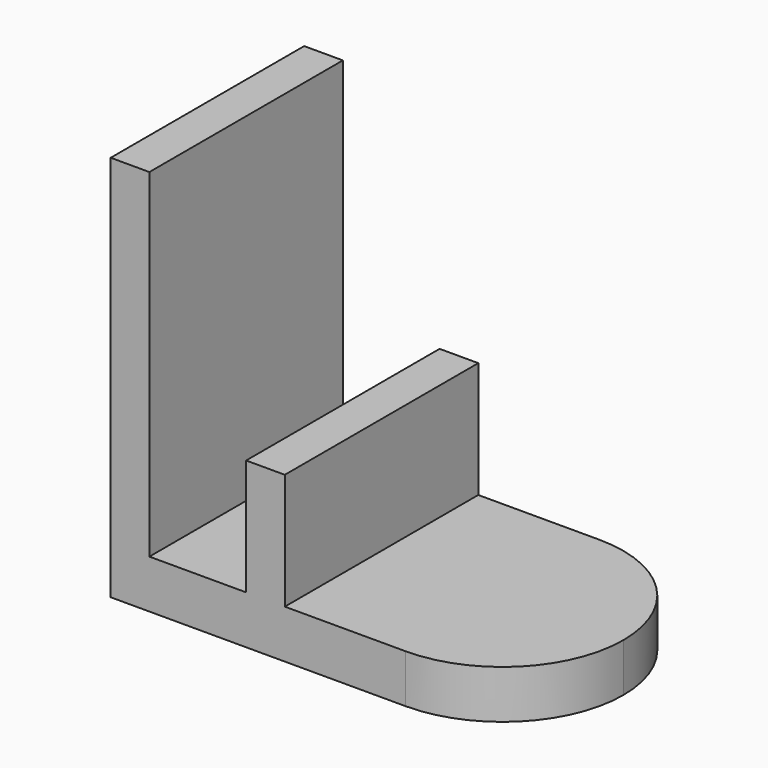
from build123d import *

# Parameters (mm, degrees)
F2_DEPTH = 50
F3_R     = 25
F4_R     = 24.99999


# Not quite as in the source:
# - a fillet or chamfer is up to 0.001 mm smaller than in the source, because OpenCascade refuses the exact size


with BuildPart() as f2:
    # F1 (on face) → F2 (new body)
    with BuildSketch(Plane.XZ):
        Polygon((8, 80), (0, 80), (0, 0), (86, 0), (86, 10), (61, 10), (36, 10), (36, 34), (28, 34), (28, 10), (8, 10), align=None)
    extrude(amount=F2_DEPTH)

    # F3
    f3_edges = [f2.edges().sort_by_distance(p)[0] for p in [
        (86, -50, 5),
    ]]
    fillet(f3_edges, radius=F3_R)

    # F4 (radius 25 in the source; OpenCascade refuses exactly that, so slightly less here)
    f4_edges = [f2.edges().sort_by_distance(p)[0] for p in [
        (86, 0, 5),
    ]]
    fillet(f4_edges, radius=F4_R)


solid = f2.part
